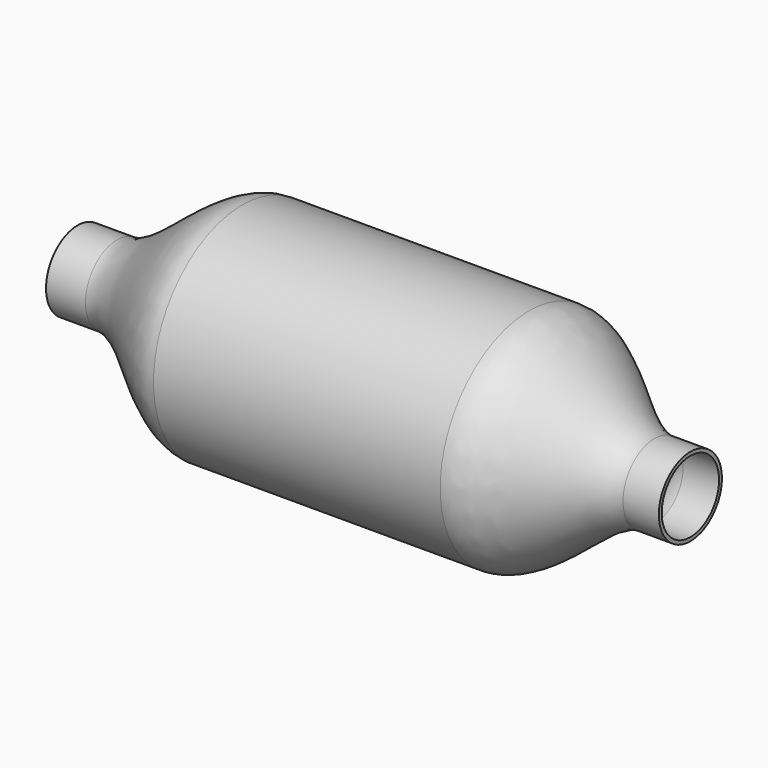
from build123d import *

# Parameters (mm, degrees)
F3_R     = 11
F4_DEPTH = 1


# Not quite as in the source:
# - the dataset's text gives a spline's control points without its knots; the knots are read off the source's solid


with BuildPart() as f1:
    # F0 (on Top) → F1 (revolve)
    with BuildSketch(Plane.XY):
        with BuildLine():
            Line((-46.5389013521, 11), (-46.5389013521, 10))
            Line((-46.5389013521, 10), (-36.5389013521, 10))
            add(Edge.make_bspline(
                [(-1.5389013521, 30), (-12.2107750812, 30), (-25.8670276231, 10), (-36.5389013521, 10)],
                knots=[0, 0, 0, 0, 40.3112887415, 40.3112887415, 40.3112887415, 40.3112887415], degree=3))
            Line((-1.5389013521, 30), (78.4610986479, 30))
            add(Edge.make_bspline(
                [(78.4610986479, 30), (89.1329723769, 30), (102.7892249188, 10), (113.4610986479, 10)],
                knots=[0, 0, 0, 0, 40.3112887415, 40.3112887415, 40.3112887415, 40.3112887415], degree=3))
            Line((113.4610986479, 10), (123.4610986479, 10))
            Line((123.4610986479, 10), (123.4610986479, 11))
            Line((123.4610986479, 11), (113.4610986479, 11))
            add(Edge.make_bspline(
                [(78.4610986479, 31), (79.2061776369, 31), (80.7033065403, 30.8254941367), (83.6998364368, 29.9006855927), (87.4597344426, 27.8678949055), (92.0213060704, 24.5338015697), (96.6028023621, 20.7668104813), (101.144353422, 17.0338015697), (105.5659363889, 13.8053949055), (109.0588459507, 11.9319355927), (111.654722973, 11.1379941367), (112.8721934207, 11), (113.4610986479, 11)],
                knots=[0, 0, 0, 0, 0.0625, 0.125, 0.25, 0.375, 0.5, 0.625, 0.75, 0.875, 0.9375, 1, 1, 1, 1], degree=3))
            Line((78.4610986479, 31), (-1.5389013521, 31))
            add(Edge.make_bspline(
                [(-1.5389013521, 31), (-2.2839803411, 31), (-3.7811092446, 30.8254941367), (-6.7776391411, 29.9006855927), (-10.5375371468, 27.8678949055), (-15.0991087747, 24.5338015697), (-19.6806050664, 20.7668104813), (-24.2221561263, 17.0338015697), (-28.6437390932, 13.8053949055), (-32.136648655, 11.9319355927), (-34.7325256772, 11.1379941367), (-35.949996125, 11), (-36.5389013521, 11)],
                knots=[0, 0, 0, 0, 0.0625, 0.125, 0.25, 0.375, 0.5, 0.625, 0.75, 0.875, 0.9375, 1, 1, 1, 1], degree=3))
            Line((-36.5389013521, 11), (-46.5389013521, 11))
        make_face()
    revolve(axis=Axis((15.9602873027, 0, 0), (1, 0, 0)))

    # F3 (on plane+point) → F4 (join)
    with BuildSketch(Plane.YZ.offset(-46.5389013521)):
        Circle(F3_R)
    extrude(amount=-F4_DEPTH)


solid = f1.part
